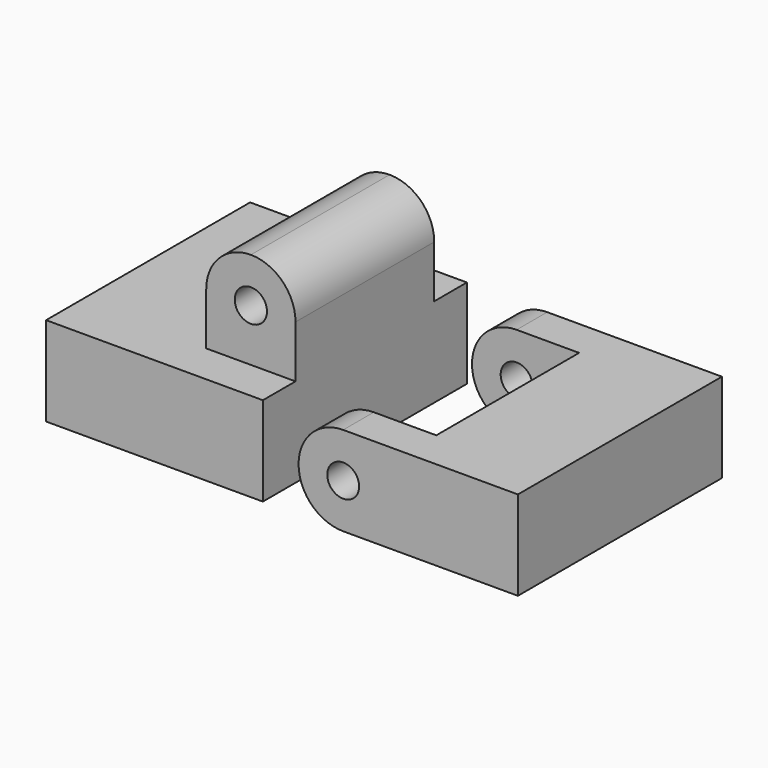
from build123d import *

# Parameters (mm, degrees)
F0_W      = 9.144
F0_H      = 3.81
F1_DEPTH  = 8.89
F3_DEPTH  = 8.89
F4_W      = 8.89
F4_H      = 17.272
F5_DEPTH  = 9.652
F6_R      = 1.60655
F7_DEPTH  = 25.4
F8_R      = 1.5875
F9_DEPTH  = 25.4
F10_R     = 4.44499
F10_2_R   = 4.44499
F11_SIZE  = 1.524
F12_DEPTH = 8.89


# Not quite as in the source:
# - a fillet or chamfer is up to 0.001 mm smaller than in the source, because OpenCascade refuses the exact size


with BuildPart() as f1:
    # F0 (on Top) → F1 (new body)
    with BuildSketch(Plane.XY):
        Polygon((-4.1064491987, 16.167118521), (-16.8064491987, 16.167118521), (-16.8064491987, 12.357118521), (-16.8064491987, -5.422881479), (-16.8064491987, -9.232881479), (-4.1064491987, -9.232881479), align=None)
        with Locations((-21.3784491987, 14.262118521)):
            Rectangle(F0_W, F0_H)
        with Locations((-21.3784491987, -7.327881479)):
            Rectangle(F0_W, F0_H)
    extrude(amount=F1_DEPTH)

    # F8 (on face) → F9 (cut)
    with BuildSketch(Plane.XZ.offset(9.232881479)):
        with Locations((-21.5054491987, 4.445)):
            Circle(F8_R)
    extrude(amount=-F9_DEPTH, mode=Mode.SUBTRACT)

    # F10#2 (radius 4.445 in the source; OpenCascade refuses exactly that, so slightly less here)
    f10_2_edges = [f1.edges().sort_by_distance(p)[0] for p in [
        (-25.950449, -7.327881, 8.89),
        (-25.950449, -7.327881, 0),
        (-25.950449, 14.262119, 0),
        (-25.950449, 14.262119, 8.89),
    ]]
    fillet(f10_2_edges, radius=F10_2_R)

    # F11
    f11_edges = [f1.edges().sort_by_distance(p)[0] for p in [
        (-16.806449, 3.467119, 8.89),
        (-16.806449, 3.467119, 0),
    ]]
    chamfer(f11_edges, length=F11_SIZE)


with BuildPart() as f3:
    # F2 (on Top) → F3 (new body)
    with BuildSketch(Plane.XY):
        Polygon((-38.3964491987, 12.103118521), (-38.3964491987, 16.167118521), (-51.0964491987, 16.167118521), (-51.0964491987, -9.232881479), (-38.3964491987, -9.232881479), (-38.3964491987, -5.168881479), (-29.5064491987, -5.168881479), (-29.5064491987, 12.103118521), align=None)
    extrude(amount=F3_DEPTH)

    # F4 (on face) → F5 (join)
    with BuildSketch(Plane.XY.offset(8.89)):
        with Locations((-33.9514491987, 3.467118521)):
            Rectangle(F4_W, F4_H)
    extrude(amount=F5_DEPTH)

    # F6 (on face) → F7 (cut)
    with BuildSketch(Plane.XZ.offset(5.168881479)):
        with Locations((-33.9514491987, 14.097)):
            Circle(F6_R)
    extrude(amount=-F7_DEPTH, mode=Mode.SUBTRACT)

    # F10 (radius 4.445 in the source; OpenCascade refuses exactly that, so slightly less here)
    f10_edges = [f3.edges().sort_by_distance(p)[0] for p in [
        (-29.506449, 3.467119, 18.542),
        (-38.396449, 3.467119, 18.542),
    ]]
    fillet(f10_edges, radius=F10_R)

    # F12 (add, through all): faces of the model
    f12_faces = [f3.faces().sort_by_distance(p)[0] for p in [
        (-38.3964491987, -7.200881479, 4.445),
        (-38.3964491987, 14.135118521, 4.445),
    ]]
    extrude(f12_faces, amount=F12_DEPTH)


solid = Compound([f1.part, f3.part])
